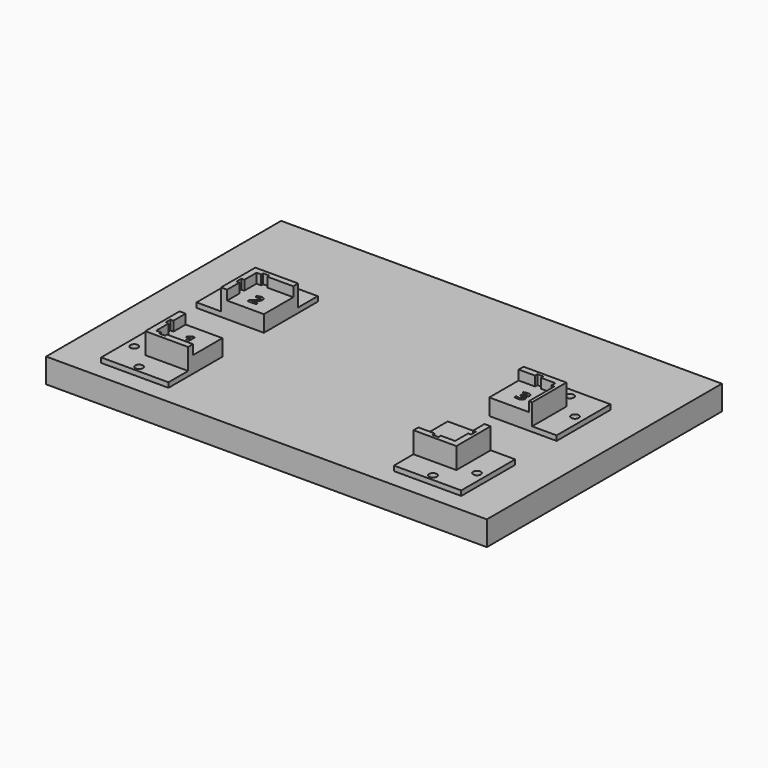
from build123d import *

# Parameters (mm, degrees)
F0_W          = 457.2
F0_H          = 304.8
F1_DEPTH      = 25.4
F3_DEPTH      = 27
F4_W          = 38.1
F4_H          = 38.1
F5_DEPTH      = 17
F4_R          = 3.96875
F6_DEPTH      = 5.08
F7_W          = 6.35
F7_H          = 2.54
F7_W_2        = 3.048
F7_H_2        = 6.35
F8_DEPTH      = 10
F9_W          = 6.35
F9_H          = 3.048
F9_W_2        = 3.048
F9_H_2        = 33.02
F9_H_3        = 6.35
F10_DEPTH     = 10
F11_TEXT_SIZE = 17.6388888889
F12_DEPTH     = 2.54


# Not quite as in the source:
# - Text() gives the source's letters only with a copy of the font that has no kerning and outlines rounded to 1/6400 em; it was checked with that copy


with BuildPart() as f1:
    # F0 (on Top) → F1 (new body)
    with BuildSketch(Plane.XY):
        Rectangle(F0_W, F0_H)
    extrude(amount=F1_DEPTH)


with BuildPart() as f3:
    # F2 (on face) → F3 (new body)
    with BuildSketch(Plane.XY.offset(25.4)):
        Polygon((-161.29, 34.75), (-161.29, -9.7), (-154.94, -9.7), (-154.94, 28.4), (-116.84, 28.4), (-116.84, 34.75), align=None)
    extrude(amount=F3_DEPTH)

    # F4 (on face) → F5 (join)
    with BuildSketch(Plane.XY.offset(25.4)):
        with Locations((-135.89, 9.35)):
            Rectangle(F4_W, F4_H)
    extrude(amount=F5_DEPTH)

    # F4 (on face) → F6 (join)
    with BuildSketch(Plane.XY.offset(25.4)):
        Polygon((-186.69, 60.15), (-186.69, -9.7), (-161.29, -9.7), (-161.29, 34.75), (-116.84, 34.75), (-116.84, 60.15), align=None)
        with Locations((-177.8, 25.4)):
            Circle(F4_R, mode=Mode.SUBTRACT)
        with Locations((-152.4, 50.8)):
            Circle(F4_R, mode=Mode.SUBTRACT)
    extrude(amount=F6_DEPTH)


with BuildPart() as f3b:
    # F2 (on face) → F3, piece 2 (new body)
    with BuildSketch(Plane.XY.offset(25.4)):
        Polygon((-116.84, -101.6), (-154.94, -101.6), (-154.94, -63.5), (-161.29, -63.5), (-161.29, -107.95), (-116.84, -107.95), align=None)
    extrude(amount=F3_DEPTH)

    # F4 (on face) → F5, piece 3 (join)
    with BuildSketch(Plane.XY.offset(25.4)):
        with Locations((-135.89, -82.55)):
            Rectangle(F4_W, F4_H)
    extrude(amount=F5_DEPTH)

    # F4 (on face) → F6, piece 2 (join)
    with BuildSketch(Plane.XY.offset(25.4)):
        Polygon((-186.69, -63.5), (-186.69, -133.35), (-116.84, -133.35), (-116.84, -107.95), (-161.29, -107.95), (-161.29, -63.5), align=None)
        with Locations((-152.4, -127)):
            Circle(F4_R, mode=Mode.SUBTRACT)
        with Locations((-177.8, -101.6)):
            Circle(F4_R, mode=Mode.SUBTRACT)
    extrude(amount=F6_DEPTH)


with BuildPart() as f3c:
    # F2 (on face) → F3, piece 3 (new body)
    with BuildSketch(Plane.XY.offset(25.4)):
        Polygon((161.41, -9.7), (161.41, 34.75), (116.96, 34.75), (116.96, 28.4), (155.06, 28.4), (155.06, -9.7), align=None)
    extrude(amount=F3_DEPTH)

    # F4 (on face) → F5, piece 2 (join)
    with BuildSketch(Plane.XY.offset(25.4)):
        with Locations((136.01, 9.35)):
            Rectangle(F4_W, F4_H)
    extrude(amount=F5_DEPTH)

    # F4 (on face) → F6, piece 3 (join)
    with BuildSketch(Plane.XY.offset(25.4)):
        Polygon((186.81, -9.7), (186.81, 60.15), (116.96, 60.15), (116.96, 34.75), (161.41, 34.75), (161.41, -9.7), align=None)
        with Locations((177.8, 25.4)):
            Circle(F4_R, mode=Mode.SUBTRACT)
        with Locations((152.4, 50.8)):
            Circle(F4_R, mode=Mode.SUBTRACT)
    extrude(amount=F6_DEPTH)


with BuildPart() as f3d:
    # F2 (on face) → F3, piece 4 (new body)
    with BuildSketch(Plane.XY.offset(25.4)):
        Polygon((161.41, -107.95), (161.41, -63.5), (155.06, -63.5), (155.06, -101.6), (116.96, -101.6), (116.96, -107.95), align=None)
    extrude(amount=F3_DEPTH)

    # F4 (on face) → F5, piece 4 (join)
    with BuildSketch(Plane.XY.offset(25.4)):
        with Locations((136.01, -82.55)):
            Rectangle(F4_W, F4_H)
    extrude(amount=F5_DEPTH)

    # F4 (on face) → F6, piece 4 (join)
    with BuildSketch(Plane.XY.offset(25.4)):
        Polygon((116.96, -133.35), (186.81, -133.35), (186.81, -63.5), (161.41, -63.5), (161.41, -107.95), (116.96, -107.95), align=None)
        with Locations((152.4, -127)):
            Circle(F4_R, mode=Mode.SUBTRACT)
        with Locations((177.8, -101.6)):
            Circle(F4_R, mode=Mode.SUBTRACT)
    extrude(amount=F6_DEPTH)


with BuildPart() as f8_tool:
    # F7 (on face) → F8 (new body, through all)
    with BuildSketch(Plane.XY.offset(52.4)):
        with Locations((-146.94, 29.67)):
            Rectangle(F7_W, F7_H)
        with Locations((-156.464, 9.35)):
            Rectangle(F7_W_2, F7_H_2)
        with Locations((-156.464, -82.55)):
            Rectangle(F7_W_2, F7_H_2)
        with Locations((-146.94, -102.87)):
            Rectangle(F7_W, F7_H)
    extrude(amount=-F8_DEPTH)


with BuildPart() as f3_1:
    add(f3.part)

    # F8: cut by f8_tool
    add(f8_tool.part, mode=Mode.SUBTRACT)


with BuildPart() as f3b_1:
    add(f3b.part)

    # F8: cut by f8_tool
    add(f8_tool.part, mode=Mode.SUBTRACT)


with BuildPart() as f10_tool:
    # F9 (on face) → F10 (new body, through all)
    with BuildSketch(Plane.XY.offset(52.4)):
        with Locations((137.06, 29.924)):
            Rectangle(F9_W, F9_H)
        with Locations((156.584, 6.81)):
            Rectangle(F9_W_2, F9_H_2)
        with Locations((156.584, -81.473)):
            Rectangle(F9_W_2, F9_H_3)
        with Locations((137.06, -103.124)):
            Rectangle(F9_W, F9_H)
    extrude(amount=-F10_DEPTH)


with BuildPart() as f3c_1:
    add(f3c.part)

    # F10: cut by f10_tool
    add(f10_tool.part, mode=Mode.SUBTRACT)


with BuildPart() as f3d_1:
    add(f3d.part)

    # F10: cut by f10_tool
    add(f10_tool.part, mode=Mode.SUBTRACT)


with BuildPart() as f12_tool:
    # F11 (on face) → F12 (new body)
    with BuildSketch(Plane.XY.offset(42.4)):
        with Locations((-142.24, -88.9)):
            Text('1', F11_TEXT_SIZE, font='Open Sans', font_style=FontStyle.BOLD, text_align=(TextAlign.LEFT, TextAlign.BOTTOM))
        with Locations((-142.24, 0)):
            Text('2', F11_TEXT_SIZE, font='Open Sans', font_style=FontStyle.BOLD, text_align=(TextAlign.LEFT, TextAlign.BOTTOM))
        with Locations((131.8290321181, 3)):
            Text('3', F11_TEXT_SIZE, font='Open Sans', font_style=FontStyle.BOLD, text_align=(TextAlign.LEFT, TextAlign.BOTTOM))
    extrude(amount=-F12_DEPTH)


with BuildPart() as f3_2:
    add(f3_1.part)

    # F12: cut by f12_tool
    add(f12_tool.part, mode=Mode.SUBTRACT)


with BuildPart() as f3b_2:
    add(f3b_1.part)

    # F12: cut by f12_tool
    add(f12_tool.part, mode=Mode.SUBTRACT)


with BuildPart() as f3c_2:
    add(f3c_1.part)

    # F12: cut by f12_tool
    add(f12_tool.part, mode=Mode.SUBTRACT)


solid = Compound([f1.part, f3d_1.part, f3_2.part, f3b_2.part, f3c_2.part])
